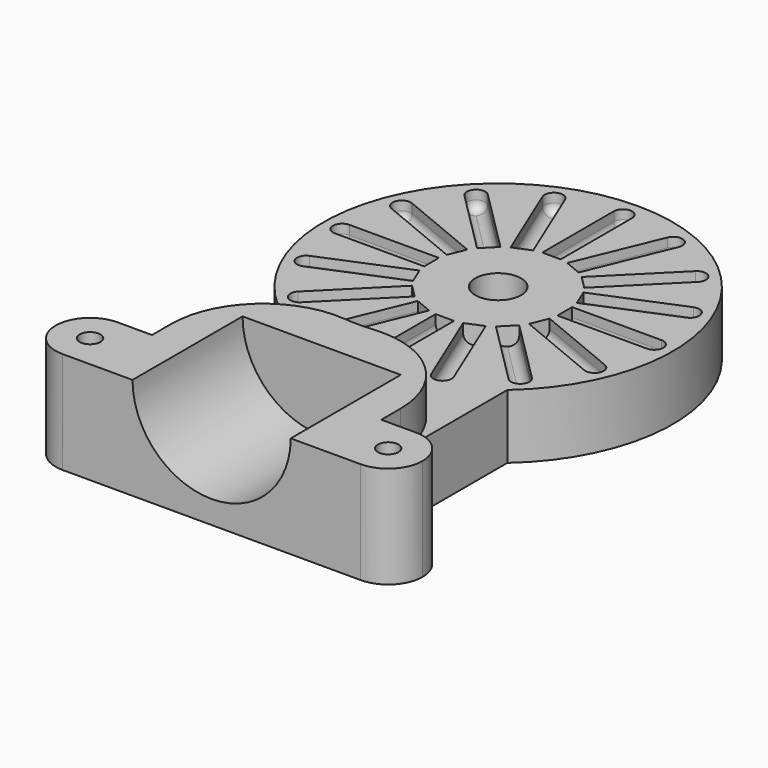
from build123d import *

# Parameters (mm, degrees)
F0_R            = 5
F1_DEPTH        = 14
F3_DEPTH        = 4
F3_COPIES_COUNT = 16
F4_R            = 1.99999
F5_R            = 2.25
F6_DEPTH        = 22.25
F7_R            = 17.25
F8_DEPTH        = 30
F9_R            = 4
F10_DEPTH       = 17
F11_S5_R        = 2.25
F11_T6_DEPTH    = 7
F11_S11_R       = 2.25
F11_T12_DEPTH   = 7
F12_R           = 20
F13_R           = 7.49999


# Not quite as in the source:
# - a fillet or chamfer that OpenCascade refuses, or shapes differently, is made with other operations: its cross-section is extruded or revolved along the edge and cut away or added
# - a fillet or chamfer is up to 0.001 mm smaller than in the source, because OpenCascade refuses the exact size
# - a pattern or mirror of a feature is missing from the dataset's text; its kind, count and spacing are read off the source's solid


with BuildPart() as f1:
    # F0 (on Top) → F1 (new body)
    with BuildSketch(Plane.XY):
        with BuildLine():
            ThreePointArc((-38.1, 0), (0, -38.1), (38.1, 0))
            ThreePointArc((38.1, 0), (0, 38.1), (-38.1, 0))
        make_face()
        Circle(F0_R, mode=Mode.SUBTRACT)
    extrude(amount=F1_DEPTH)

    # F2 (on face) → F3 (cut)
    with BuildSketch(Plane.XY.offset(14)):
        with BuildLine():
            Line((14.525, -2), (34.025, -2))
            ThreePointArc((34.025, -2), (36.025, 0), (34.025, 2))
            Line((34.025, 2), (14.525, 2))
            Line((14.525, 2), (14.525, -2))
        make_face()
    f3 = extrude(amount=-F3_DEPTH, mode=Mode.SUBTRACT)

    # F3_copies: F3 ×16 about axis
    f3_copies_axis = Axis((0, 0, 0), (0, 0, 1))
    for i in range(1, F3_COPIES_COUNT):
        add(f3.rotate(f3_copies_axis, i * 360 / F3_COPIES_COUNT), mode=Mode.SUBTRACT)

    # F4 (radius 2 in the source; OpenCascade refuses exactly that, so slightly less here)
    f4_edges = [f1.edges().sort_by_distance(p)[0] for p in [
        (24.275, 2, 10),
        (-11.137399, -21.661809, 10),
        (-13.786171, -33.28276, 10),
        (-7.441881, -23.192543, 10),
        (-2, -24.275, 10),
        (0, -36.025, 10),
        (2, -24.275, 10),
        (-23.192543, -7.441881, 10),
        (-33.28276, -13.786171, 10),
        (-21.661809, -11.137399, 10),
        (-18.579231, -15.750804, 10),
        (-25.473522, -25.473522, 10),
        (-15.750804, -18.579231, 10),
        (7.441881, -23.192543, 10),
        (13.786171, -33.28276, 10),
        (11.137399, -21.661809, 10),
        (15.750804, -18.579231, 10),
        (25.473522, -25.473522, 10),
        (18.579231, -15.750804, 10),
        (21.661809, -11.137399, 10),
        (33.28276, -13.786171, 10),
        (23.192543, -7.441881, 10),
        (-24.275, 2, 10),
        (-36.025, 0, 10),
        (-24.275, -2, 10),
        (-21.661809, 11.137399, 10),
        (-33.28276, 13.786171, 10),
        (-23.192543, 7.441881, 10),
        (-15.750804, 18.579231, 10),
        (-25.473522, 25.473522, 10),
        (-18.579231, 15.750804, 10),
        (-7.441881, 23.192543, 10),
        (-13.786171, 33.28276, 10),
        (-11.137399, 21.661809, 10),
        (18.579231, 15.750804, 10),
        (25.473522, 25.473522, 10),
        (15.750804, 18.579231, 10),
        (24.275, -2, 10),
        (36.025, 0, 10),
        (23.192543, 7.441881, 10),
        (33.28276, 13.786171, 10),
        (21.661809, 11.137399, 10),
        (2, 24.275, 10),
        (0, 36.025, 10),
        (-2, 24.275, 10),
        (11.137399, 21.661809, 10),
        (13.786171, 33.28276, 10),
        (7.441881, 23.192543, 10),
    ]]
    fillet(f4_edges, radius=F4_R)

    # F5 (on Top) → F6 (join)
    with BuildSketch(Plane.XY):
        with BuildLine():
            ThreePointArc((0, -38.1), (-13.345477259, -35.6862471651), (-25, -28.7508260751))
            Line((-25, -28.7508260751), (-25, -63.1))
            Line((-25, -63.1), (-40, -63.1))
            Line((-40, -63.1), (-40, -78.1))
            Line((-40, -78.1), (-25, -78.1))
            Line((-25, -78.1), (0, -78.1))
            Line((0, -78.1), (25, -78.1))
            Line((25, -78.1), (40, -78.1))
            Line((40, -78.1), (40, -63.1))
            Line((40, -63.1), (25, -63.1))
            Line((25, -63.1), (25, -28.7508260751))
            ThreePointArc((25, -28.7508260751), (13.345477259, -35.6862471651), (0, -38.1))
        make_face()
        with Locations((-32.5, -70.6)):
            Circle(F5_R, mode=Mode.SUBTRACT)
        with Locations((32.5, -70.6)):
            Circle(F5_R, mode=Mode.SUBTRACT)
    extrude(amount=F6_DEPTH)

    # F7 (on face) → F8 (cut)
    with BuildSketch(Plane.XZ.offset(78.1)):
        with Locations((0, 22.25)):
            Circle(F7_R)
    extrude(amount=-F8_DEPTH, mode=Mode.SUBTRACT)

    # F9 (on Top) → F10 (cut)
    with BuildSketch(Plane.XY):
        with Locations((-32.5, -70.6)):
            Circle(F9_R)
        with Locations((32.5, -70.6)):
            Circle(F9_R)
    extrude(amount=F10_DEPTH, mode=Mode.SUBTRACT)

    # F11: chamfer of 2.5 on 2 edges, made by hand


with BuildPart() as f11_tool2:
    # F11_s3 → F11_t4 (revolve)
    with BuildSketch(Plane.XZ.offset(70.6)):
        Polygon((-28.5, 14.5), (-31, 17), (-28.5, 17), align=None)
    revolve(axis=Axis((-32.5, -70.6, 17), (0, 0, 1)))

    # F11_s5 → F11_t6 (cut, symmetric)
    with BuildSketch(Plane.XY.offset(15.8)):
        with Locations((-32.5, -70.6)):
            Circle(F11_S5_R)
    extrude(amount=F11_T6_DEPTH, both=True, mode=Mode.SUBTRACT)


with BuildPart() as f1_1:
    add(f1.part)

    # F11_t1: union F11_tool2
    add(f11_tool2.part)


with BuildPart() as f11_tool8:
    # F11_s9 → F11_t10 (revolve)
    with BuildSketch(Plane.XZ.offset(70.6)):
        Polygon((36.5, 14.5), (34, 17), (36.5, 17), align=None)
    revolve(axis=Axis((32.5, -70.6, 17), (0, 0, 1)))

    # F11_s11 → F11_t12 (cut, symmetric)
    with BuildSketch(Plane.XY.offset(15.8)):
        with Locations((32.5, -70.6)):
            Circle(F11_S11_R)
    extrude(amount=F11_T12_DEPTH, both=True, mode=Mode.SUBTRACT)


with BuildPart() as f1_2:
    add(f1_1.part)

    # F11_t7: union F11_tool8
    add(f11_tool8.part)

    # F12
    f12_edges = [f1_2.edges().sort_by_distance(p)[0] for p in [
        (25, -28.750826, 18.125),
        (-25, -28.750826, 18.125),
    ]]
    fillet(f12_edges, radius=F12_R)

    # F13 (radius 7.5 in the source; OpenCascade refuses exactly that, so slightly less here)
    f13_edges = [f1_2.edges().sort_by_distance(p)[0] for p in [
        (-40, -63.1, 11.125),
        (-40, -78.1, 11.125),
        (40, -78.1, 11.125),
        (40, -63.1, 11.125),
    ]]
    fillet(f13_edges, radius=F13_R)


solid = f1_2.part
